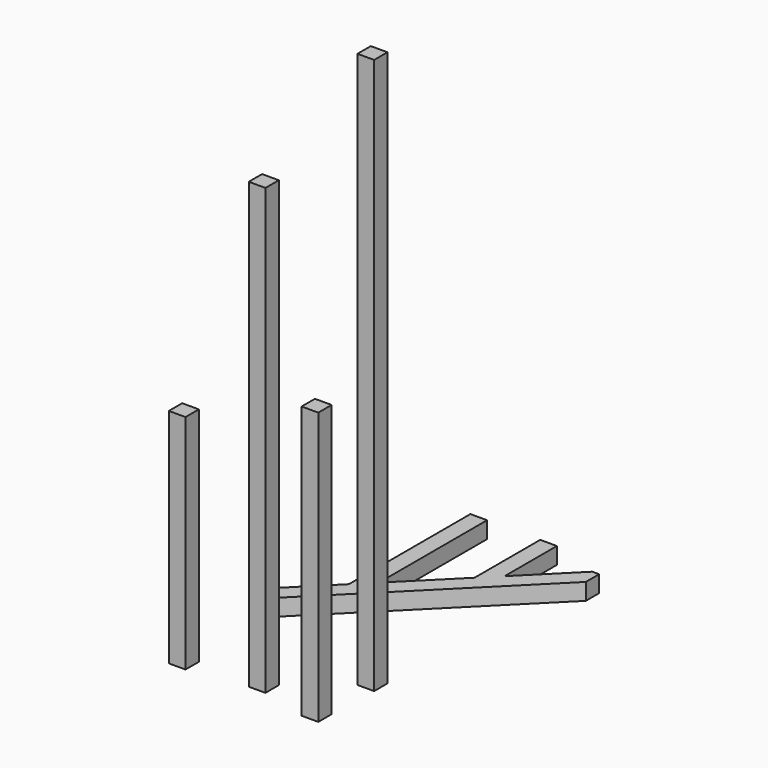
from build123d import *

# Parameters (mm, degrees)
F0_W     = 9
F0_H     = 9
F1_DEPTH = 300
F2_W     = 9
F2_H     = 9
F3_DEPTH = 120
F4_W     = 9
F4_H     = 9
F5_DEPTH = 240
F6_W     = 9
F6_H     = 5.27208
F7_DEPTH = 9
F8_W     = 9
F8_H     = 9
F9_DEPTH = 147


# Not quite as in the source:
# - a feature names something its author has since deleted; it is built from what else it names


with BuildPart() as f1:
    # F0 (on Top) → F1 (new body)
    with BuildSketch(Plane.XY):
        Rectangle(F0_W, F0_H)
    extrude(amount=F1_DEPTH)


with BuildPart() as f3:
    # F2 (on Top) → F3 (new body)
    with BuildSketch(Plane.XY):
        with Locations((-74.4131075144, -34.275306195)):
            Rectangle(F2_W, F2_H)
    extrude(amount=F3_DEPTH)


with BuildPart() as f5:
    # F4 (on Top) → F5 (new body)
    with BuildSketch(Plane.XY):
        with Locations((-34.7862875015, -29.8701094389)):
            Rectangle(F4_W, F4_H)
    extrude(amount=F5_DEPTH)


with BuildPart() as f7:
    # F6 (on Top) → F7 (new body)
    with BuildSketch(Plane.XY):
        Polygon((-45.0111036971, 60.6276517883), (-54.0111036971, 51.6276517883), (-79.2943466264, 26.3444088591), (-79.2943466264, 22.6164888591), (-70.294344565, 22.6164888591), (22.7056533736, 115.6164867977), (22.7056533736, 124.6164888591), (18.9777333736, 124.6164888591), (-7.3252493367, 98.3135061488), (-16.3252493367, 89.3135061488), align=None)
        Polygon((-45.0111036971, 128.3444088591), (-54.0111036971, 128.3444088591), (-54.0111036971, 51.6276517883), (-45.0111036971, 60.6276517883), align=None)
        with Locations((-49.5111036971, 130.9804488591)):
            Rectangle(F6_W, F6_H)
        Polygon((-7.3252493367, 128.3444088591), (-16.3252493367, 128.3444088591), (-16.3252493367, 89.3135061488), (-7.3252493367, 98.3135061488), align=None)
        with Locations((-11.8252493367, 130.9804488591)):
            Rectangle(F6_W, F6_H)
    extrude(amount=F7_DEPTH)


with BuildPart() as f9:
    # F8 (on Top) → F9 (new body)
    with BuildSketch(Plane.XY):
        with Locations((-0.8312522359, -36.646684438)):
            Rectangle(F8_W, F8_H)
    extrude(amount=F9_DEPTH)


solid = Compound([f1.part, f3.part, f5.part, f7.part, f9.part])
